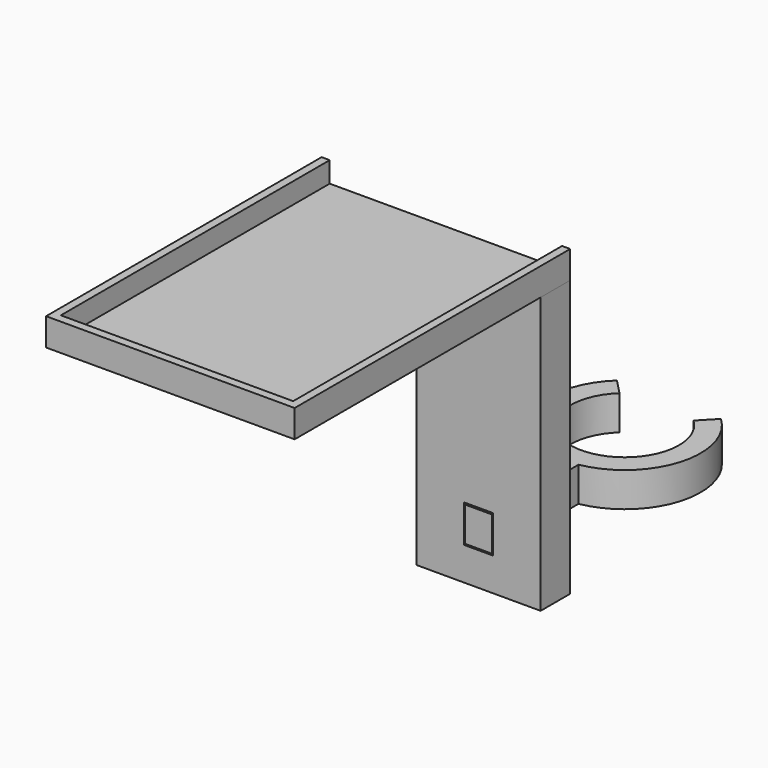
from build123d import *

# Parameters (mm, degrees)
F1_DEPTH      = 12.7
F2_W          = 17.8625439294
F2_H          = 13.6123597622
F2_W_2        = 9.9653182551
F3_DEPTH      = 76.2
F3_DEPTH_BACK = 25.4
F4_W          = 10.7960565947
F4_H          = 13.7910920894
F5_DEPTH      = 12.7
F6_W          = 91.5096271783
F6_H          = 126.8072500825
F7_DEPTH      = 2.54
F8_W          = 85.5362936854
F8_H          = 3.070384264
F9_DEPTH      = 7.62


with BuildPart() as f1:
    # F0 (on Top) → F1 (new body)
    with BuildSketch(Plane.XY):
        with BuildLine():
            ThreePointArc((-19.1484129168, 47.8582315663), (-26.7988757538, 19.5681342696), (-4.9826591276, 0))
            Line((-4.9826591276, 0), (-4.9826591276, -39.7654548287))
            Line((-4.9826591276, -39.7654548287), (4.9826591276, -39.7654548287))
            Line((4.9826591276, -39.7654548287), (4.9826591276, 0))
            ThreePointArc((4.9826591276, 0), (26.7988757538, 19.5681342696), (19.1484129168, 47.8582315663))
            Line((19.1484129168, 47.8582315663), (13.6314762534, 42.1173290091))
            ThreePointArc((13.6314762534, 42.1173290091), (18.5958954805, 20.1749282956), (0, 7.5136851253))
            ThreePointArc((0, 7.5136851253), (-18.5958954805, 20.1749282956), (-13.6314762534, 42.1173290091))
            Line((-13.6314762534, 42.1173290091), (-19.1484129168, 47.8582315663))
        make_face()
    extrude(amount=F1_DEPTH)


with BuildPart() as f3:
    # F2 (on face) → F3 (new body, two sides)
    with BuildSketch(Plane.XY.offset(12.7)) as f3_sk:
        with Locations((-13.9139310922, -32.9592749476)):
            Rectangle(F2_W, F2_H)
        with Locations((0, -32.9592749476)):
            Rectangle(F2_W_2, F2_H)
        with Locations((13.9139310922, -32.9592749476)):
            Rectangle(F2_W, F2_H)
    extrude(amount=F3_DEPTH)
    extrude(f3_sk.sketch, amount=-F3_DEPTH_BACK)

    # F4 (on face) → F5 (cut)
    with BuildSketch(Plane.XZ.offset(39.7654548287)):
        with Locations((-0.0001469161, 6.4032858354)):
            Rectangle(F4_W, F4_H)
    extrude(amount=-F5_DEPTH, mode=Mode.SUBTRACT)


with BuildPart() as f7:
    # F6 (on face) → F7 (new body)
    with BuildSketch(Plane.XY.offset(88.9)):
        with Locations((-22.9096105322, -89.5567201078)):
            Rectangle(F6_W, F6_H)
    extrude(amount=F7_DEPTH)

    # F8 (on face) → F9 (join)
    with BuildSketch(Plane.XY.offset(91.44)):
        Polygon((-65.6880363822, -26.1530950665), (-68.6644241214, -26.1530950665), (-68.6644241214, -152.960345149), (-65.6880363822, -152.960345149), (-65.6880363822, -149.889960885), align=None)
        with Locations((-22.9198895395, -151.425153017)):
            Rectangle(F8_W, F8_H)
        Polygon((19.8482573032, -26.1530950665), (19.8482573032, -149.889960885), (19.8482573032, -152.960345149), (22.8452030569, -152.960345149), (22.8452030569, -26.1530950665), align=None)
    extrude(amount=F9_DEPTH)


solid = Compound([f1.part, f3.part, f7.part])
